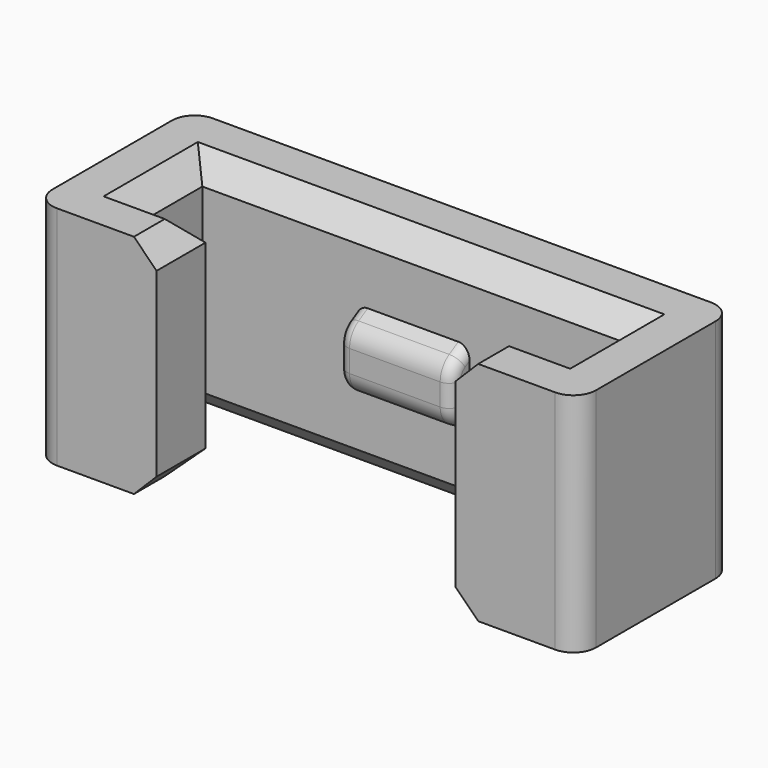
from build123d import *

# Parameters (mm, degrees)
F1_DEPTH    = 10
F2_W        = 5
F2_H        = 3.4
F3_DEPTH    = 1
F4_T4_DEPTH = 10.6915886602
F4_T9_DEPTH = 10.6915886602
F5_R        = 1
F6_R        = 0.5
F7_SIZE     = 1
F8_R        = 1


# Not quite as in the source:
# - a fillet or chamfer that OpenCascade refuses, or shapes differently, is made with other operations: its cross-section is extruded or revolved along the edge and cut away or added


with BuildPart() as f1:
    # F0 (on Top) → F1 (new body)
    with BuildSketch(Plane.XY):
        Polygon((-6.6, -5.9), (-9.3, -5.9), (-9.3, -2.7), (0, -2.7), (9.3, -2.7), (9.3, -5.9), (6.6, -5.9), (6.6, -8.6), (12, -8.6), (12, 0), (0, 0), (-12, 0), (-12, -8.6), (-6.6, -8.6), align=None)
    extrude(amount=F1_DEPTH)

    # F2 (on face) → F3 (join)
    with BuildSketch(Plane.XZ.offset(2.7)):
        with Locations((0, 5)):
            Rectangle(F2_W, F2_H)
    extrude(amount=F3_DEPTH)

    # F4: chamfer of 1.1 x 0.6350852961 on 2 edges, made by hand


with BuildPart() as f4_tool2:
    # F4_s3 → F4_t4 (new body)
    with BuildSketch(Plane.YZ.offset(5.3457943301)):
        Polygon((-2.6, 6.7), (-3.7, 6.0649147039), (-3.7, 6.7), align=None)
    extrude(amount=-F4_T4_DEPTH)

    split(bisect_by=Plane.XZ.offset(2.7), keep=Keep.TOP)


with BuildPart() as f1_1:
    add(f1.part)

    # F4_t1: cut F4_tool2
    add(f4_tool2.part, mode=Mode.SUBTRACT)


with BuildPart() as f4_tool7:
    # F4_s8 → F4_t9 (new body)
    with BuildSketch(Plane.YZ.offset(-5.3457943301)):
        Polygon((-2.6, 3.3), (-3.7, 3.9350852961), (-3.7, 3.3), align=None)
    extrude(amount=F4_T9_DEPTH)

    split(bisect_by=Plane.XZ.offset(2.7), keep=Keep.TOP)


with BuildPart() as f1_2:
    add(f1_1.part)

    # F4_t6: cut F4_tool7
    add(f4_tool7.part, mode=Mode.SUBTRACT)

    # F5
    f5_edges = [f1_2.edges().sort_by_distance(p)[0] for p in [
        (0, -3.7, 3.935085),
        (0, -3.7, 6.064915),
    ]]
    fillet(f5_edges, radius=F5_R)

    # F6
    f6_edges = [f1_2.edges().sort_by_distance(p)[0] for p in [
        (2.5, -3.566025, 4.012436),
        (2.5, -3.566025, 5.987564),
        (-2.5, -3.566025, 4.012436),
        (-2.5, -3.566025, 5.987564),
        (2.5, -2.95, 6.497927),
        (-2.5, -2.95, 6.497927),
        (2.5, -3.7, 5),
        (2.5, -2.95, 3.502073),
        (-2.5, -2.95, 3.502073),
        (-2.5, -3.7, 5),
    ]]
    fillet(f6_edges, radius=F6_R)

    # F7
    f7_edges = [f1_2.edges().sort_by_distance(p)[0] for p in [
        (-9.3, -4.3, 0),
        (0, -2.7, 0),
        (-7.95, -5.9, 0),
        (-6.6, -7.25, 0),
        (9.3, -4.3, 0),
        (7.95, -5.9, 0),
        (6.6, -7.25, 0),
        (-9.3, -4.3, 10),
        (-7.95, -5.9, 10),
        (-6.6, -7.25, 10),
        (0, -2.7, 10),
        (9.3, -4.3, 10),
        (7.95, -5.9, 10),
        (6.6, -7.25, 10),
    ]]
    chamfer(f7_edges, length=F7_SIZE)

    # F8
    f8_edges = [f1_2.edges().sort_by_distance(p)[0] for p in [
        (-12, -8.6, 5),
        (12, -8.6, 5),
        (-12, 0, 5),
        (12, 0, 5),
    ]]
    fillet(f8_edges, radius=F8_R)


solid = f1_2.part
